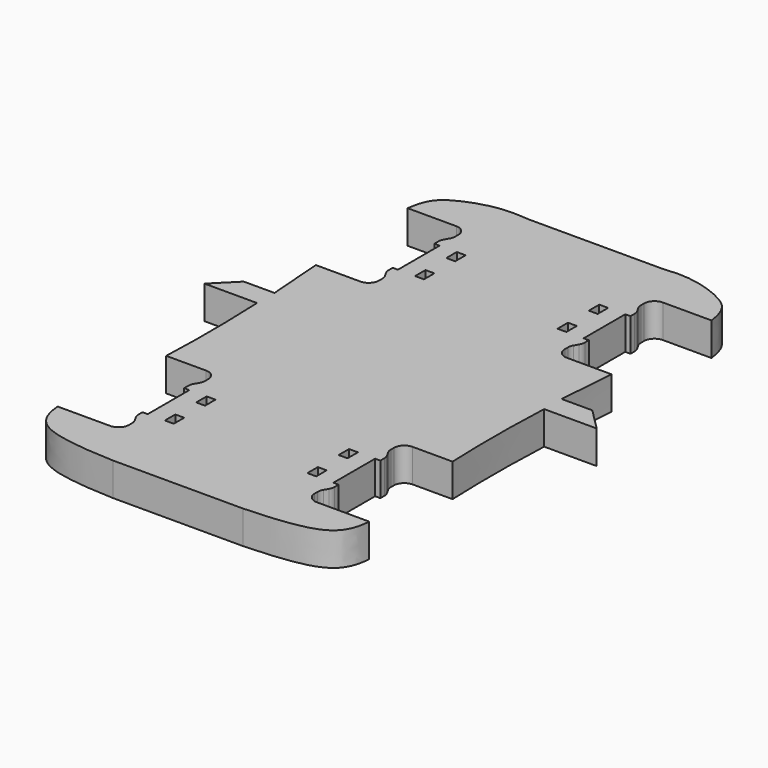
from build123d import *

# Parameters (mm, degrees)
F1_W     = 1.7
F1_H     = 2.5
F2_DEPTH = 6.35


# Not quite as in the source:
# - a feature names something its author has since deleted; it is built from what else it names


with BuildPart() as f2:
    # F1 (on Top) → F2 (new body)
    with BuildSketch(Plane.XY):
        with BuildLine():
            add(Edge.make_bspline(
                [(-28.3662502266, 18.5), (-28.0282859794, 14.509768022), (-27.7307294384, 11.0425580188), (-27.5446102023, 7.5721158646)],
                knots=[0.8198316729, 0.8198316729, 0.8198316729, 0.8198316729, 1, 1, 1, 1], degree=3))
            Line((-27.5446102023, 7.5721158646), (-33.4338024259, 7.5721158646))
            Line((-33.4338024259, 7.5721158646), (-37.6275889575, 3.3783284016))
            Line((-37.6275889575, 3.3783284016), (-27.5446102023, 3.3783284016))
            add(Edge.make_bspline(
                [(-27.5446102023, 3.3783284016), (-27.1626822342, -4.8739274421), (-27.2042266074, -12.4503556404), (-27.4753266797, -18.5)],
                knots=[0, 0, 0, 0, 0.2300812655, 0.2300812655, 0.2300812655, 0.2300812655], degree=3))
            Line((-27.4753266797, -18.5), (-19.8166404351, -18.5))
            ThreePointArc((-19.8166404351, -18.5), (-18.4024268727, -19.0857864376), (-17.8166404351, -20.5))
            Line((-17.8166404351, -20.5), (-17.8166404351, -21.2320508076))
            ThreePointArc((-17.8166404351, -21.2320508076), (-17.8847887825, -21.7496888978), (-18.0845896275, -22.2320508076))
            Line((-18.0845896275, -22.2320508076), (-18.5486912426, -23.0358983849))
            ThreePointArc((-18.5486912426, -23.0358983849), (-18.7484920877, -23.5182602947), (-18.8166404351, -24.0358983849))
            Line((-18.8166404351, -24.0358983849), (-18.8166404351, -25))
            Line((-18.8166404351, -25), (-17.8166404351, -25))
            Line((-17.8166404351, -25), (-17.8166404351, -30))
            Line((-17.8166404351, -30), (-17.8166404351, -35))
            Line((-17.8166404351, -35), (-18.8166404351, -35))
            Line((-18.8166404351, -35), (-18.8166404351, -35.9641016151))
            ThreePointArc((-18.8166404351, -35.9641016151), (-18.7484920877, -36.4817397053), (-18.5486912426, -36.9641016151))
            Line((-18.5486912426, -36.9641016151), (-18.0845896275, -37.7679491924))
            ThreePointArc((-18.0845896275, -37.7679491924), (-17.8847887825, -38.2503111022), (-17.8166404351, -38.7679491924))
            Line((-17.8166404351, -38.7679491924), (-17.8166404351, -39.5))
            ThreePointArc((-17.8166404351, -39.5), (-18.4024268727, -40.9142135624), (-19.8166404351, -41.5))
            Line((-19.8166404351, -41.5), (-29.8822661517, -41.5))
            add(Edge.make_bspline(
                [(-29.8822661517, -41.5), (-29.7521644168, -43.7295834581), (-28.3532415217, -48.2000718925), (-19.0537112462, -49.6748582384), (-14.8830911746, -49.9236971311), (-12.5, -50)],
                knots=[0.5930961397, 0.5930961397, 0.5930961397, 0.5930961397, 0.7144689073, 0.865116052, 1, 1, 1, 1], degree=3))
            Line((-12.5, -50), (12.5, -50))
            add(Edge.make_bspline(
                [(29.8822661517, -41.5), (29.7521644168, -43.7295834581), (28.3532415217, -48.2000718925), (19.0537112462, -49.6748582384), (14.8830911746, -49.9236971311), (12.5, -50)],
                knots=[0.5930961397, 0.5930961397, 0.5930961397, 0.5930961397, 0.7144689073, 0.865116052, 1, 1, 1, 1], degree=3))
            Line((29.8822661517, -41.5), (19.8166404351, -41.5))
            ThreePointArc((19.8166404351, -41.5), (18.4024268727, -40.9142135624), (17.8166404351, -39.5))
            Line((17.8166404351, -39.5), (17.8166404351, -38.7679491924))
            ThreePointArc((17.8166404351, -38.7679491924), (17.8847887825, -38.2503111022), (18.0845896275, -37.7679491924))
            Line((18.0845896275, -37.7679491924), (18.5486912426, -36.9641016151))
            ThreePointArc((18.5486912426, -36.9641016151), (18.7484920877, -36.4817397053), (18.8166404351, -35.9641016151))
            Line((18.8166404351, -35.9641016151), (18.8166404351, -35))
            Line((18.8166404351, -35), (17.8166404351, -35))
            Line((17.8166404351, -35), (17.8166404351, -30))
            Line((17.8166404351, -30), (17.8166404351, -25))
            Line((17.8166404351, -25), (18.8166404351, -25))
            Line((18.8166404351, -25), (18.8166404351, -24.0358983849))
            ThreePointArc((18.8166404351, -24.0358983849), (18.7484920877, -23.5182602947), (18.5486912426, -23.0358983849))
            Line((18.5486912426, -23.0358983849), (18.0845896275, -22.2320508076))
            ThreePointArc((18.0845896275, -22.2320508076), (17.8847887825, -21.7496888978), (17.8166404351, -21.2320508076))
            Line((17.8166404351, -21.2320508076), (17.8166404351, -20.5))
            ThreePointArc((17.8166404351, -20.5), (18.4024268727, -19.0857864376), (19.8166404351, -18.5))
            Line((19.8166404351, -18.5), (27.4753266797, -18.5))
            add(Edge.make_bspline(
                [(27.5446102023, 3.3783284016), (27.1626822342, -4.8739274421), (27.2042266074, -12.4503556404), (27.4753266797, -18.5)],
                knots=[0, 0, 0, 0, 0.2300812655, 0.2300812655, 0.2300812655, 0.2300812655], degree=3))
            Line((27.5446102023, 3.3783284016), (37.6275889575, 3.3783284016))
            Line((37.6275889575, 3.3783284016), (33.4338024259, 7.5721158646))
            Line((33.4338024259, 7.5721158646), (27.5446102023, 7.5721158646))
            add(Edge.make_bspline(
                [(28.3662502266, 18.5), (28.0282859794, 14.509768022), (27.7307294384, 11.0425580188), (27.5446102023, 7.5721158646)],
                knots=[0.8198316729, 0.8198316729, 0.8198316729, 0.8198316729, 1, 1, 1, 1], degree=3))
            Line((28.3662502266, 18.5), (19.8166404351, 18.5))
            ThreePointArc((19.8166404351, 18.5), (18.4024268727, 19.0857864376), (17.8166404351, 20.5))
            Line((17.8166404351, 20.5), (17.8166404351, 21.2320508076))
            ThreePointArc((17.8166404351, 21.2320508076), (17.8847887825, 21.7496888978), (18.0845896275, 22.2320508076))
            Line((18.0845896275, 22.2320508076), (18.5486912426, 23.0358983849))
            ThreePointArc((18.5486912426, 23.0358983849), (18.7484920877, 23.5182602947), (18.8166404351, 24.0358983849))
            Line((18.8166404351, 24.0358983849), (18.8166404351, 25))
            Line((18.8166404351, 25), (17.8166404351, 25))
            Line((17.8166404351, 25), (17.8166404351, 30))
            Line((17.8166404351, 30), (17.8166404351, 35))
            Line((17.8166404351, 35), (18.8166404351, 35))
            Line((18.8166404351, 35), (18.8166404351, 35.9641016151))
            ThreePointArc((18.8166404351, 35.9641016151), (18.7484920877, 36.4817397053), (18.5486912426, 36.9641016151))
            Line((18.5486912426, 36.9641016151), (18.0845896275, 37.7679491924))
            ThreePointArc((18.0845896275, 37.7679491924), (17.8847887825, 38.2503111022), (17.8166404351, 38.7679491924))
            Line((17.8166404351, 38.7679491924), (17.8166404351, 39.5))
            ThreePointArc((17.8166404351, 39.5), (18.4024268727, 40.9142135624), (19.8166404351, 41.5))
            Line((19.8166404351, 41.5), (29.1458233545, 41.5))
            add(Edge.make_bspline(
                [(12.5, 50), (14.4284018661, 50.1560744709), (18.4905820055, 50.4849939867), (25.8883531216, 47.9554177216), (28.4554923405, 45.4024265549), (29.0501411907, 42.2200084299), (29.1458233545, 41.5)],
                knots=[0, 0, 0, 0, 0.1539827529, 0.3243842758, 0.4690112538, 0.5065425276, 0.5065425276, 0.5065425276, 0.5065425276], degree=3))
            Line((12.5, 50), (-12.5, 50))
            add(Edge.make_bspline(
                [(-12.5, 50), (-14.4284018661, 50.1560744709), (-18.4905820055, 50.4849939867), (-25.8883531216, 47.9554177216), (-28.4554923405, 45.4024265549), (-29.0501411907, 42.2200084299), (-29.1458233545, 41.5)],
                knots=[0, 0, 0, 0, 0.1539827529, 0.3243842758, 0.4690112538, 0.5065425276, 0.5065425276, 0.5065425276, 0.5065425276], degree=3))
            Line((-29.1458233545, 41.5), (-19.8166404351, 41.5))
            ThreePointArc((-19.8166404351, 41.5), (-18.4024268727, 40.9142135624), (-17.8166404351, 39.5))
            Line((-17.8166404351, 39.5), (-17.8166404351, 38.7679491924))
            ThreePointArc((-17.8166404351, 38.7679491924), (-17.8847887825, 38.2503111022), (-18.0845896275, 37.7679491924))
            Line((-18.0845896275, 37.7679491924), (-18.5486912426, 36.9641016151))
            ThreePointArc((-18.5486912426, 36.9641016151), (-18.7484920877, 36.4817397053), (-18.8166404351, 35.9641016151))
            Line((-18.8166404351, 35.9641016151), (-18.8166404351, 35))
            Line((-18.8166404351, 35), (-17.8166404351, 35))
            Line((-17.8166404351, 35), (-17.8166404351, 30))
            Line((-17.8166404351, 30), (-17.8166404351, 25))
            Line((-17.8166404351, 25), (-18.8166404351, 25))
            Line((-18.8166404351, 25), (-18.8166404351, 24.0358983849))
            ThreePointArc((-18.8166404351, 24.0358983849), (-18.7484920877, 23.5182602947), (-18.5486912426, 23.0358983849))
            Line((-18.5486912426, 23.0358983849), (-18.0845896275, 22.2320508076))
            ThreePointArc((-18.0845896275, 22.2320508076), (-17.8847887825, 21.7496888978), (-17.8166404351, 21.2320508076))
            Line((-17.8166404351, 21.2320508076), (-17.8166404351, 20.5))
            ThreePointArc((-17.8166404351, 20.5), (-18.4024268727, 19.0857864376), (-19.8166404351, 18.5))
            Line((-19.8166404351, 18.5), (-28.3662502266, 18.5))
        make_face()
        with Locations((-13.6666404351, -33.75)):
            Rectangle(F1_W, F1_H, mode=Mode.SUBTRACT)
        with Locations((-13.6666404351, -26.25)):
            Rectangle(F1_W, F1_H, mode=Mode.SUBTRACT)
        with Locations((13.6666404351, -33.75)):
            Rectangle(F1_W, F1_H, mode=Mode.SUBTRACT)
        with Locations((13.6666404351, -26.25)):
            Rectangle(F1_W, F1_H, mode=Mode.SUBTRACT)
        with Locations((-13.6666404351, 26.25)):
            Rectangle(F1_W, F1_H, mode=Mode.SUBTRACT)
        with Locations((-13.6666404351, 33.75)):
            Rectangle(F1_W, F1_H, mode=Mode.SUBTRACT)
        with Locations((13.6666404351, 26.25)):
            Rectangle(F1_W, F1_H, mode=Mode.SUBTRACT)
        with Locations((13.6666404351, 33.75)):
            Rectangle(F1_W, F1_H, mode=Mode.SUBTRACT)
    extrude(amount=F2_DEPTH)


solid = f2.part
